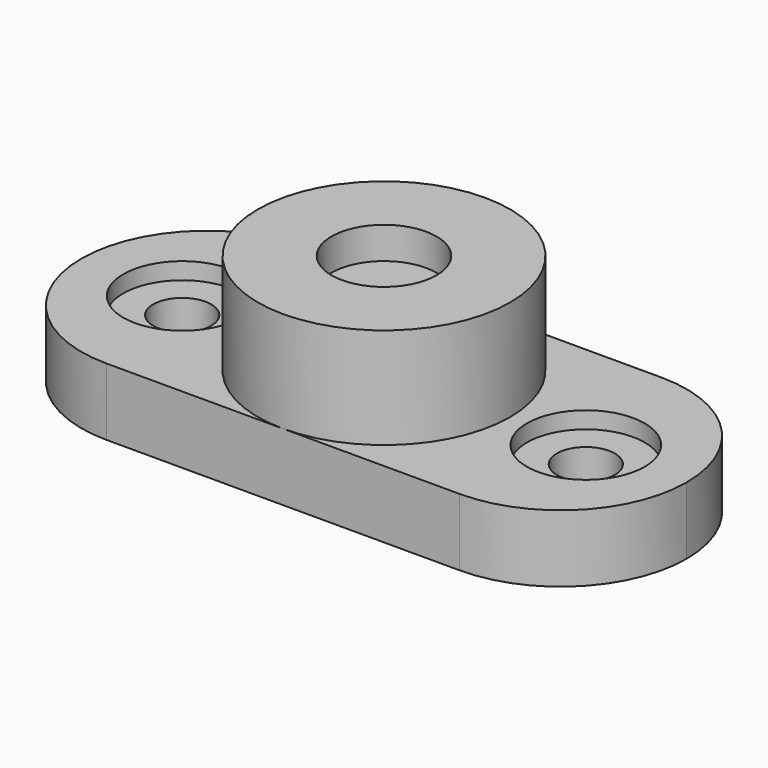
from build123d import *

# Parameters (mm, degrees)
F0_W      = 36
F0_H      = 15
F1_DEPTH  = 4
F2_R      = 7.5
F3_DEPTH  = 6
F4_R      = 7.49999
F6_DEPTH  = 8
F7_R      = 1.725
F8_DEPTH  = 4
F7_R_2    = 3.5
F9_DEPTH  = 1
F10_R     = 3.125
F11_DEPTH = 2
F12_R     = 3.2
F13_DEPTH = 0.1
F14_R     = 7
F15_DEPTH = 2.6
F17_DEPTH = 0.2


# Not quite as in the source:
# - a fillet or chamfer is up to 0.001 mm smaller than in the source, because OpenCascade refuses the exact size


with BuildPart() as f1:
    # F0 (on Top) → F1 (new body)
    with BuildSketch(Plane.XY):
        Rectangle(F0_W, F0_H)
    extrude(amount=F1_DEPTH)

    # F2 (on face) → F3 (join)
    with BuildSketch(Plane.XY.offset(4)):
        Circle(F2_R)
    extrude(amount=F3_DEPTH)

    # F4 (radius 7.5 in the source; OpenCascade refuses exactly that, so slightly less here)
    f4_edges = [f1.edges().sort_by_distance(p)[0] for p in [
        (-18, -7.5, 2),
        (-18, 7.5, 2),
        (18, -7.5, 2),
        (18, 7.5, 2),
    ]]
    fillet(f4_edges, radius=F4_R)

    # F5 (on face) → F6 (cut)
    with BuildSketch(Plane(origin=(0, 0, 0), x_dir=(1, 0, 0), z_dir=(0, 0, -1))):
        Polygon((2.8867513459, 5), (-2.8867513459, 5), (-5.7735026919, 0), (-2.8867513459, -5), (2.8867513459, -5), (5.7735026919, 0), align=None)
    extrude(amount=-F6_DEPTH, mode=Mode.SUBTRACT)

    # F7 (on face) → F8 (cut, through all)
    with BuildSketch(Plane.XY.offset(4)):
        with Locations((12, 0)):
            Circle(F7_R)
        with Locations((-12, 0)):
            Circle(F7_R)
    extrude(amount=-F8_DEPTH, mode=Mode.SUBTRACT)

    # F7 (on face) → F9 (cut)
    with BuildSketch(Plane.XY.offset(4)):
        with Locations((-12, 0)):
            Circle(F7_R_2)
        with Locations((-12, 0)):
            Circle(F7_R, mode=Mode.SUBTRACT)
        with Locations((12, 0)):
            Circle(F7_R_2)
        with Locations((12, 0)):
            Circle(F7_R, mode=Mode.SUBTRACT)
    extrude(amount=-F9_DEPTH, mode=Mode.SUBTRACT)

    # F10 (on face) → F11 (cut, through all)
    with BuildSketch(Plane.XY.offset(10)):
        Circle(F10_R)
    extrude(amount=-F11_DEPTH, mode=Mode.SUBTRACT)

    # F12 (on face) → F13 (join)
    with BuildSketch(Plane(origin=(0, 0, 8), x_dir=(1, 0, 0), z_dir=(0, 0, -1))):
        Circle(F12_R)
    extrude(amount=-F13_DEPTH)

    # F14 (on face) → F15 (cut)
    with BuildSketch(Plane(origin=(0, 0, 0), x_dir=(1, 0, 0), z_dir=(0, 0, -1))):
        Circle(F14_R)
    extrude(amount=-F15_DEPTH, mode=Mode.SUBTRACT)

    # F16 (on face) → F17 (join)
    with BuildSketch(Plane(origin=(0, 0, 2.6), x_dir=(1, 0, 0), z_dir=(0, 0, -1))):
        Polygon((2.8867513459, 5), (-2.8867513459, 5), (-5.7735026919, 0), (-2.8867513459, -5), (2.8867513459, -5), (5.7735026919, 0), align=None)
    extrude(amount=-F17_DEPTH)


solid = f1.part
